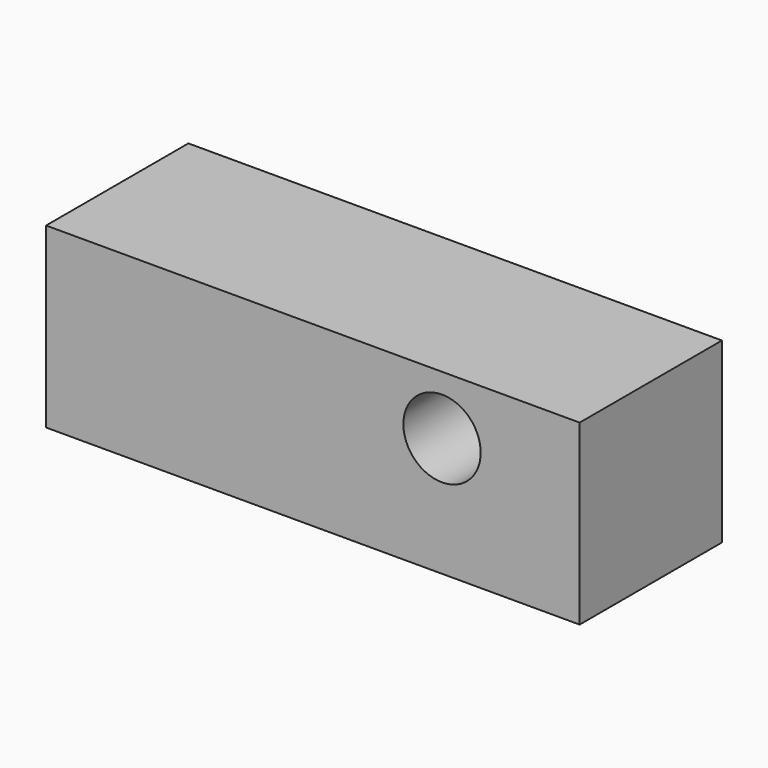
from build123d import *

# Parameters (mm, degrees)
F0_W     = 150
F0_H     = 50
F1_DEPTH = 50
F4_R     = 10.8716166344
F5_DEPTH = 61


# Not quite as in the source:
# - the program builds the solid bodies; features that only make, move or delete a surface that nothing else refers to are left out


with BuildPart() as f1:
    # F0 (on Front) → F1 (new body)
    with BuildSketch(Plane.XZ):
        with Locations((4.0709814262, 25)):
            Rectangle(F0_W, F0_H)
    extrude(amount=F1_DEPTH)

    # F4 (on face) → F5 (cut)
    with BuildSketch(Plane(origin=(0, 0, 0), x_dir=(-1, 0, 0), z_dir=(0, 1, 0))):
        with Locations((-40.3841286898, 33.4967449307)):
            Circle(F4_R)
    extrude(amount=-F5_DEPTH, mode=Mode.SUBTRACT)


solid = f1.part
